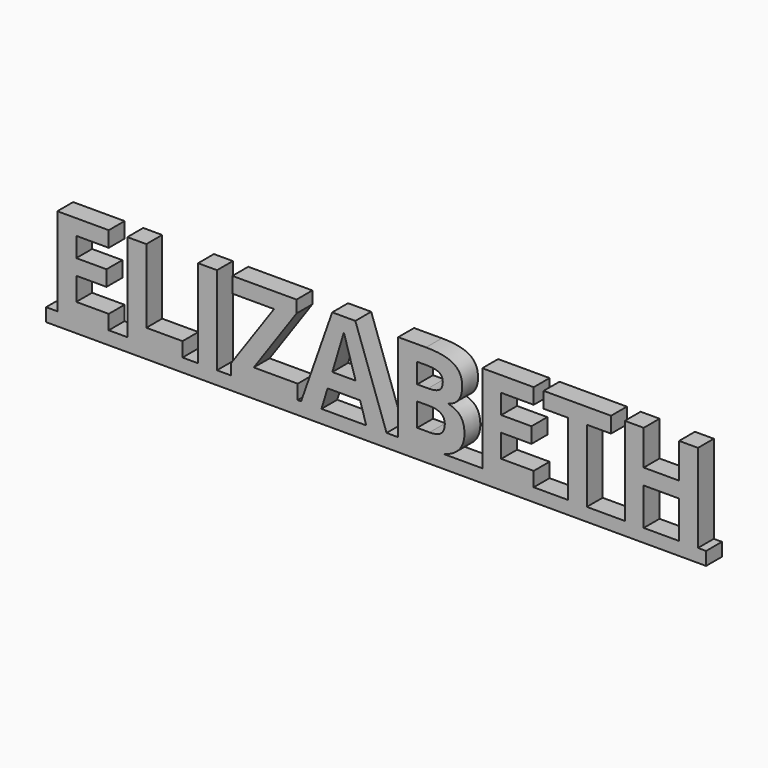
from build123d import *

# Parameters (mm, degrees)
F0_W         = 100
F0_H         = 2
F2_DEPTH     = 3
F1_TEXT_SIZE = 18.9545387235
F3_DEPTH     = 3


# Not quite as in the source:
# - Text() gives the source's letters only with a copy of the font that has no kerning and outlines rounded to 1/6400 em; it was checked with that copy


with BuildPart() as f2:
    # F0 (on Front) → F2 (new body)
    with BuildSketch(Plane.XZ):
        with Locations((0, -0.8186144405)):
            Rectangle(F0_W, F0_H)
    extrude(amount=F2_DEPTH)

    # F1 (on Front) → F3 (join)
    with BuildSketch(Plane.XZ):
        with Locations((-50, 0)):
            Text('ELIZABETH', F1_TEXT_SIZE, font='Open Sans', font_style=FontStyle.BOLD, text_align=(TextAlign.LEFT, TextAlign.BOTTOM))
    extrude(amount=F3_DEPTH)


solid = f2.part
